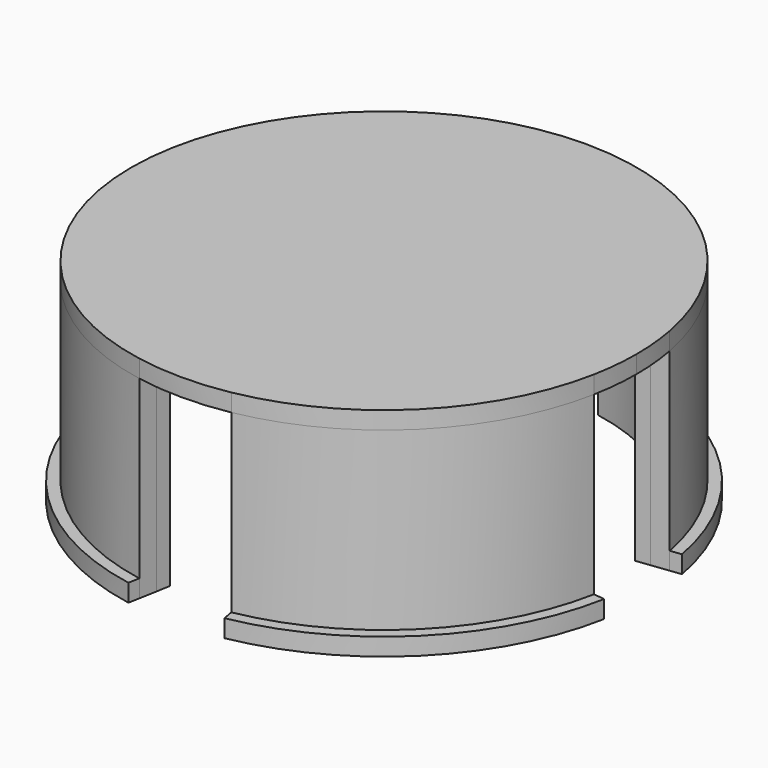
from build123d import *

# Parameters (mm, degrees)
F1_DEPTH = 1
F2_DEPTH = 11
F3_DEPTH = 10


with BuildPart() as f1:
    # F0 (on Top) → F1 (new body)
    with BuildSketch(Plane.XY):
        with BuildLine():
            ThreePointArc((12.3109959605, -2.4885695612), (12.4975939537, -1.250498048), (12.56, 0))
            ThreePointArc((12.56, 0), (12.499849565, 1.227746249), (12.3199743866, 2.4437330282))
            ThreePointArc((12.3199743866, 2.4437330282), (8.8241351782, 8.9380220607), (2.2855528975, 12.3502974844))
            ThreePointArc((2.2855528975, 12.3502974844), (0.0100228873, 12.5599960009), (-2.2658389037, 12.3539294988))
            ThreePointArc((-2.2658389037, 12.3539294988), (-8.8620220769, 8.9004586797), (-12.3440076572, 2.3192832854))
            ThreePointArc((-12.3440076572, 2.3192832854), (-12.559977123, 0.023972266), (-12.3527709674, -2.2721464362))
            ThreePointArc((-12.3527709674, -2.2721464362), (-8.8868925427, -8.8756262277), (-2.2878147001, -12.3498786997))
            ThreePointArc((-2.2878147001, -12.3498786997), (0.0002376292, -12.5599999978), (2.2882820061, -12.3497921222))
            ThreePointArc((2.2882820061, -12.3497921222), (8.8088397015, -8.9530968449), (12.3109959605, -2.4885695612))
        make_face()
        with BuildLine():
            ThreePointArc((12.3199743866, 2.4437330282), (12.499849565, 1.227746249), (12.56, 0))
            ThreePointArc((12.56, 0), (12.4975939537, -1.250498048), (12.3109959605, -2.4885695612))
            Line((12.3109959605, -2.4885695612), (13.1075011071, -2.5855424186))
            Line((13.1075011071, -2.5855424186), (14.1026028651, -2.7066940036))
            ThreePointArc((14.1026028651, -2.7066940036), (14.2955058872, -1.3594526209), (14.36, 0))
            ThreePointArc((14.36, 0), (14.2978344087, 1.334740133), (14.1118758743, 2.657923872))
            Line((14.1118758743, 2.657923872), (13.1166017889, 2.5389560617))
            Line((13.1166017889, 2.5389560617), (12.3199743866, 2.4437330282))
        make_face()
        with BuildLine():
            ThreePointArc((2.2855528975, 12.3502974844), (8.8241351782, 8.9380220607), (12.3199743866, 2.4437330282))
            Line((12.3199743866, 2.4437330282), (13.1166017889, 2.5389560617))
            Line((13.1166017889, 2.5389560617), (14.1118758743, 2.657923872))
            ThreePointArc((14.1118758743, 2.657923872), (10.136505033, 10.1715714477), (2.6091735777, 14.1209706905))
            Line((2.6091735777, 14.1209706905), (2.4293843449, 13.1372635399))
            Line((2.4293843449, 13.1372635399), (2.2855528975, 12.3502974844))
        make_face()
        with BuildLine():
            Line((13.1075011071, -2.5855424186), (12.3109959605, -2.4885695612))
            ThreePointArc((12.3109959605, -2.4885695612), (8.8088397015, -8.9530968449), (2.2882820061, -12.3497921222))
            Line((2.2882820061, -12.3497921222), (2.4340324524, -13.1364030853))
            Line((2.4340324524, -13.1364030853), (2.6162205102, -14.1196667893))
            ThreePointArc((2.6162205102, -14.1196667893), (10.1214500303, -10.1865523748), (14.1026028651, -2.7066940036))
            Line((14.1026028651, -2.7066940036), (13.1075011071, -2.5855424186))
        make_face()
        with BuildLine():
            ThreePointArc((-2.2658389037, 12.3539294988), (0.0100228873, 12.5599960009), (2.2855528975, 12.3502974844))
            Line((2.2855528975, 12.3502974844), (2.4293843449, 13.1372635399))
            Line((2.4293843449, 13.1372635399), (2.6091735777, 14.1209706905))
            ThreePointArc((2.6091735777, 14.1209706905), (-0.0077642493, 14.359997901), (-2.624442069, 14.118140948))
            Line((-2.624442069, 14.118140948), (-2.4252208949, 13.1380372835))
            Line((-2.4252208949, 13.1380372835), (-2.2658389037, 12.3539294988))
        make_face()
        with BuildLine():
            Line((2.4340324524, -13.1364030853), (2.2882820061, -12.3497921222))
            ThreePointArc((2.2882820061, -12.3497921222), (0.0002376292, -12.5599999978), (-2.2878147001, -12.3498786997))
            Line((-2.2878147001, -12.3498786997), (-2.431047805, -13.136955882))
            Line((-2.431047805, -13.136955882), (-2.6100890312, -14.1208015087))
            ThreePointArc((-2.6100890312, -14.1208015087), (0.0031177966, -14.3599996615), (2.6162205102, -14.1196667893))
            Line((2.6162205102, -14.1196667893), (2.4340324524, -13.1364030853))
        make_face()
        with BuildLine():
            ThreePointArc((-12.3440076572, 2.3192832854), (-8.8620220769, 8.9004586797), (-2.2658389037, 12.3539294988))
            Line((-2.2658389037, 12.3539294988), (-2.4252208949, 13.1380372835))
            Line((-2.4252208949, 13.1380372835), (-2.624442069, 14.118140948))
            ThreePointArc((-2.624442069, 14.118140948), (-10.146271601, 10.1618291955), (-14.1141033231, 2.6460701775))
            Line((-14.1141033231, 2.6460701775), (-13.1307172202, 2.4645219739))
            Line((-13.1307172202, 2.4645219739), (-12.3440076572, 2.3192832854))
        make_face()
        with BuildLine():
            Line((-2.431047805, -13.136955882), (-2.2878147001, -12.3498786997))
            ThreePointArc((-2.2878147001, -12.3498786997), (-8.8868925427, -8.8756262277), (-12.3527709674, -2.2721464362))
            Line((-12.3527709674, -2.2721464362), (-14.1224720777, -2.601034874))
            ThreePointArc((-14.1224720777, -2.601034874), (-10.1573080166, -10.1507976955), (-2.6100890312, -14.1208015087))
            Line((-2.6100890312, -14.1208015087), (-2.431047805, -13.136955882))
        make_face()
        with BuildLine():
            ThreePointArc((-12.3527709674, -2.2721464362), (-12.559977123, 0.023972266), (-12.3440076572, 2.3192832854))
            Line((-12.3440076572, 2.3192832854), (-13.1307172202, 2.4645219739))
            Line((-13.1307172202, 2.4645219739), (-14.1141033231, 2.6460701775))
            ThreePointArc((-14.1141033231, 2.6460701775), (-14.3599817356, 0.0229031363), (-14.1224720777, -2.601034874))
            Line((-14.1224720777, -2.601034874), (-12.3527709674, -2.2721464362))
        make_face()
    extrude(amount=F1_DEPTH)

    # F0 (on Top) → F2 (join)
    with BuildSketch(Plane.XY):
        with BuildLine():
            ThreePointArc((2.2855528975, 12.3502974844), (8.8241351782, 8.9380220607), (12.3199743866, 2.4437330282))
            Line((12.3199743866, 2.4437330282), (13.1166017889, 2.5389560617))
            Line((13.1166017889, 2.5389560617), (14.1118758743, 2.657923872))
            ThreePointArc((14.1118758743, 2.657923872), (10.136505033, 10.1715714477), (2.6091735777, 14.1209706905))
            Line((2.6091735777, 14.1209706905), (2.4293843449, 13.1372635399))
            Line((2.4293843449, 13.1372635399), (2.2855528975, 12.3502974844))
        make_face()
        with BuildLine():
            Line((13.1075011071, -2.5855424186), (12.3109959605, -2.4885695612))
            ThreePointArc((12.3109959605, -2.4885695612), (8.8088397015, -8.9530968449), (2.2882820061, -12.3497921222))
            Line((2.2882820061, -12.3497921222), (2.4340324524, -13.1364030853))
            Line((2.4340324524, -13.1364030853), (2.6162205102, -14.1196667893))
            ThreePointArc((2.6162205102, -14.1196667893), (10.1214500303, -10.1865523748), (14.1026028651, -2.7066940036))
            Line((14.1026028651, -2.7066940036), (13.1075011071, -2.5855424186))
        make_face()
        with BuildLine():
            ThreePointArc((-12.3440076572, 2.3192832854), (-8.8620220769, 8.9004586797), (-2.2658389037, 12.3539294988))
            Line((-2.2658389037, 12.3539294988), (-2.4252208949, 13.1380372835))
            Line((-2.4252208949, 13.1380372835), (-2.624442069, 14.118140948))
            ThreePointArc((-2.624442069, 14.118140948), (-10.146271601, 10.1618291955), (-14.1141033231, 2.6460701775))
            Line((-14.1141033231, 2.6460701775), (-13.1307172202, 2.4645219739))
            Line((-13.1307172202, 2.4645219739), (-12.3440076572, 2.3192832854))
        make_face()
        with BuildLine():
            ThreePointArc((2.6091735777, 14.1209706905), (10.136505033, 10.1715714477), (14.1118758743, 2.657923872))
            Line((14.1118758743, 2.657923872), (14.7487280331, 2.7340485374))
            ThreePointArc((14.7487280331, 2.7340485374), (10.6030739469, 10.6101283158), (2.7242386681, 14.7505431656))
            Line((2.7242386681, 14.7505431656), (2.6091735777, 14.1209706905))
        make_face()
        with BuildLine():
            Line((-2.431047805, -13.136955882), (-2.2878147001, -12.3498786997))
            ThreePointArc((-2.2878147001, -12.3498786997), (-8.8868925427, -8.8756262277), (-12.3527709674, -2.2721464362))
            Line((-12.3527709674, -2.2721464362), (-14.1224720777, -2.601034874))
            ThreePointArc((-14.1224720777, -2.601034874), (-10.1573080166, -10.1507976955), (-2.6100890312, -14.1208015087))
            Line((-2.6100890312, -14.1208015087), (-2.431047805, -13.136955882))
        make_face()
        with BuildLine():
            Line((14.7393400257, -2.7842154385), (14.1026028651, -2.7066940036))
            ThreePointArc((14.1026028651, -2.7066940036), (10.1214500303, -10.1865523748), (2.6162205102, -14.1196667893))
            Line((2.6162205102, -14.1196667893), (2.7328208672, -14.7489555599))
            ThreePointArc((2.7328208672, -14.7489555599), (10.5880995986, -10.6250716181), (14.7393400257, -2.7842154385))
        make_face()
        with BuildLine():
            ThreePointArc((-14.1141033231, 2.6460701775), (-10.146271601, 10.1618291955), (-2.624442069, 14.118140948))
            Line((-2.624442069, 14.118140948), (-2.7519420936, 14.7453997814))
            ThreePointArc((-2.7519420936, 14.7453997814), (-10.6028895523, 10.6103125845), (-14.7434702232, 2.7622609899))
            Line((-14.7434702232, 2.7622609899), (-14.1141033231, 2.6460701775))
        make_face()
        with BuildLine():
            ThreePointArc((-2.6100890312, -14.1208015087), (-10.1573080166, -10.1507976955), (-14.1224720777, -2.601034874))
            Line((-14.1224720777, -2.601034874), (-14.7516989871, -2.717972957))
            ThreePointArc((-14.7516989871, -2.717972957), (-10.6090110951, -10.6041917931), (-2.7246753784, -14.750462504))
            Line((-2.7246753784, -14.750462504), (-2.6100890312, -14.1208015087))
        make_face()
    extrude(amount=-F2_DEPTH)

    # F0 (on Top) → F3 (cut)
    with BuildSketch(Plane.XY):
        with BuildLine():
            ThreePointArc((-14.1141033231, 2.6460701775), (-10.146271601, 10.1618291955), (-2.624442069, 14.118140948))
            Line((-2.624442069, 14.118140948), (-2.7519420936, 14.7453997814))
            ThreePointArc((-2.7519420936, 14.7453997814), (-10.6028895523, 10.6103125845), (-14.7434702232, 2.7622609899))
            Line((-14.7434702232, 2.7622609899), (-14.1141033231, 2.6460701775))
        make_face()
        with BuildLine():
            ThreePointArc((2.6091735777, 14.1209706905), (10.136505033, 10.1715714477), (14.1118758743, 2.657923872))
            Line((14.1118758743, 2.657923872), (14.7487280331, 2.7340485374))
            ThreePointArc((14.7487280331, 2.7340485374), (10.6030739469, 10.6101283158), (2.7242386681, 14.7505431656))
            Line((2.7242386681, 14.7505431656), (2.6091735777, 14.1209706905))
        make_face()
        with BuildLine():
            Line((14.7393400257, -2.7842154385), (14.1026028651, -2.7066940036))
            ThreePointArc((14.1026028651, -2.7066940036), (10.1214500303, -10.1865523748), (2.6162205102, -14.1196667893))
            Line((2.6162205102, -14.1196667893), (2.7328208672, -14.7489555599))
            ThreePointArc((2.7328208672, -14.7489555599), (10.5880995986, -10.6250716181), (14.7393400257, -2.7842154385))
        make_face()
        with BuildLine():
            ThreePointArc((-2.6100890312, -14.1208015087), (-10.1573080166, -10.1507976955), (-14.1224720777, -2.601034874))
            Line((-14.1224720777, -2.601034874), (-14.7516989871, -2.717972957))
            ThreePointArc((-14.7516989871, -2.717972957), (-10.6090110951, -10.6041917931), (-2.7246753784, -14.750462504))
            Line((-2.7246753784, -14.750462504), (-2.6100890312, -14.1208015087))
        make_face()
    extrude(amount=-F3_DEPTH, mode=Mode.SUBTRACT)


solid = f1.part
